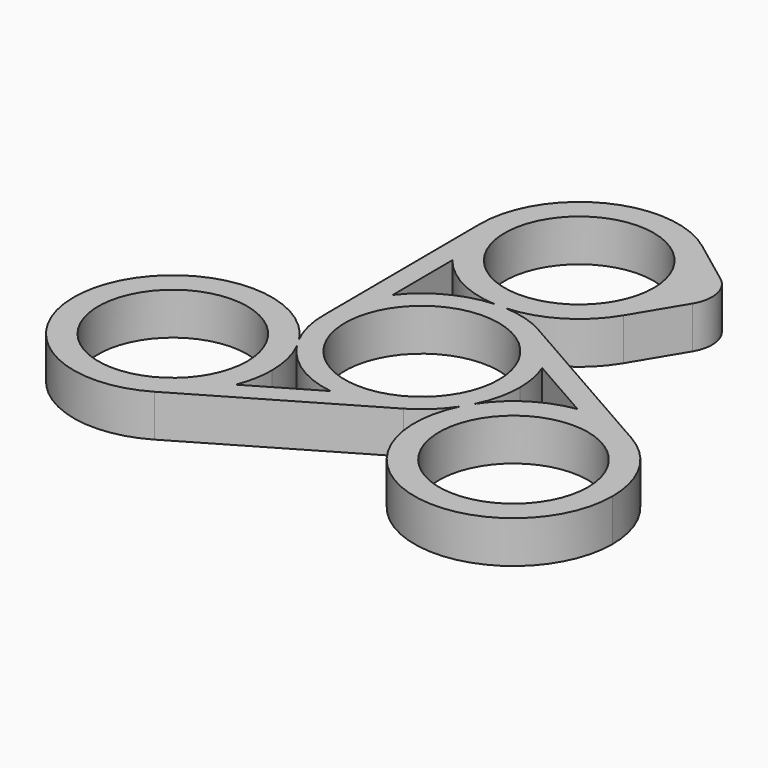
from build123d import *

# Parameters (mm, degrees)
F0_R     = 10.95
F0_R_2   = 10.6
F1_DEPTH = 6
F2_R     = 5


with BuildPart() as f1:
    # F0 (on Top) → F1 (new body)
    with BuildSketch(Plane.XY):
        with BuildLine():
            ThreePointArc((12.4777984827, -6.2375512043), (13.5769618994, -3.2044665053), (13.95, 0))
            ThreePointArc((13.95, 0), (13.6931728351, 2.6644920167), (12.932147999, 5.2308745094))
            ThreePointArc((12.932147999, 5.2308745094), (10.5018317529, 9.1822671401), (6.9101799774, 12.118247096))
            ThreePointArc((6.9101799774, 12.118247096), (3.977530702, 13.3709292689), (0.8370214411, 13.9248660714))
            ThreePointArc((0.8370214411, 13.9248660714), (0, 13.9), (-0.8370214411, 13.9248660714))
            ThreePointArc((-0.8370214411, 13.9248660714), (-6.4912873033, 12.3476997512), (-10.9961438792, 8.5841318599))
            ThreePointArc((-10.9961438792, 8.5841318599), (-13.2029923977, 4.5037197676), (-13.9497998232, -0.0747321429))
            ThreePointArc((-13.9497998232, -0.0747321429), (-13.5683297701, -3.2408220022), (-12.4777984827, -6.2375512043))
            ThreePointArc((-12.4777984827, -6.2375512043), (-12.0377531126, -6.95), (-11.6407770416, -7.6873148672))
            ThreePointArc((-11.6407770416, -7.6873148672), (-7.4477777849, -11.7954697264), (-1.9360037904, -13.8150059473))
            ThreePointArc((-1.9360037904, -13.8150059473), (2.7011607312, -13.6859866544), (7.0396198458, -12.0435149532))
            ThreePointArc((7.0396198458, -12.0435149532), (9.5907990681, -10.1301072667), (11.6407770416, -7.6873148672))
            ThreePointArc((11.6407770416, -7.6873148672), (12.0377531126, -6.95), (12.4777984827, -6.2375512043))
        make_face()
        Circle(F0_R, mode=Mode.SUBTRACT)
        with BuildLine():
            ThreePointArc((6.9101799774, 12.118247096), (10.5018317529, 9.1822671401), (12.932147999, 5.2308745094))
            Line((12.932147999, 5.2308745094), (22.1940121838, -0.0505121414))
            ThreePointArc((22.1940121838, -0.0505121414), (26.8561983982, -0.1431962176), (31.2331942939, -1.7514491718))
            Line((31.2331942939, -1.7514491718), (6.9101799774, 12.118247096))
        make_face()
        with BuildLine():
            ThreePointArc((22.1940121838, -0.0505121414), (16.67528741, -2.1065879373), (12.4777984827, -6.2375512043))
            ThreePointArc((12.4777984827, -6.2375512043), (12.0810543828, -6.975), (11.6407770416, -7.6873148672))
            ThreePointArc((11.6407770416, -7.6873148672), (21.0054007386, -27.7219144642), (38.348711306, -14))
            ThreePointArc((38.348711306, -14), (36.4407416974, -6.9173172501), (31.2331942939, -1.7514491718))
            ThreePointArc((31.2331942939, -1.7514491718), (26.8561983982, -0.1431962176), (22.1940121838, -0.0505121414))
        make_face()
        with Locations((24.248711306, -14)):
            Circle(F0_R_2, mode=Mode.SUBTRACT)
        with BuildLine():
            ThreePointArc((11.6407770416, -7.6873148672), (12.0810543828, -6.975), (12.4777984827, -6.2375512043))
            ThreePointArc((12.4777984827, -6.2375512043), (12.0377531126, -6.95), (11.6407770416, -7.6873148672))
        make_face()
        with BuildLine():
            ThreePointArc((-0.8370214411, 13.9248660714), (0, 13.9), (0.8370214411, 13.9248660714))
            ThreePointArc((0.8370214411, 13.9248660714), (0, 13.95), (-0.8370214411, 13.9248660714))
        make_face()
        with BuildLine():
            ThreePointArc((-0.8370214411, 13.9248660714), (0, 13.95), (0.8370214411, 13.9248660714))
            ThreePointArc((0.8370214411, 13.9248660714), (7.3062558034, 15.940620823), (12.0881437953, 20.7414340546))
            ThreePointArc((12.0881437953, 20.7414340546), (13.5877302651, 24.2338897729), (14.1, 28))
            ThreePointArc((14.1, 28), (12.6120042357, 34.3045498776), (8.4620781334, 39.2784411008))
            ThreePointArc((8.4620781334, 39.2784411008), (-6.338309536, 40.5950717436), (-14.0997976707, 27.9244642857))
            ThreePointArc((-14.0997976707, 27.9244642857), (-13.3040875478, 23.329747917), (-11.0532609603, 19.2458340121))
            ThreePointArc((-11.0532609603, 19.2458340121), (-6.5132847974, 15.4945163569), (-0.8370214411, 13.9248660714))
        make_face()
        with Locations((0, 28)):
            Circle(F0_R_2, mode=Mode.SUBTRACT)
        with BuildLine():
            Line((-17.1333966231, -26.1730151139), (7.0396198458, -12.0435149532))
            ThreePointArc((7.0396198458, -12.0435149532), (2.7011607312, -13.6859866544), (-1.9360037904, -13.8150059473))
            Line((-1.9360037904, -13.8150059473), (-11.1407508896, -19.1953222924))
            ThreePointArc((-11.1407508896, -19.1953222924), (-13.5521107613, -23.1865519531), (-17.1333966231, -26.1730151139))
        make_face()
        with BuildLine():
            ThreePointArc((14.1, 28), (13.5877302651, 24.2338897729), (12.0881437953, 20.7414340546))
            Line((12.0881437953, 20.7414340546), (18.6356199511, 31.6453555542))
            Line((18.6356199511, 31.6453555542), (8.4620781334, 39.2784411008))
            ThreePointArc((8.4620781334, 39.2784411008), (12.6120042357, 34.3045498776), (14.1, 28))
        make_face()
        with BuildLine():
            ThreePointArc((-12.4777984827, -6.2375512043), (-37.9792640143, -10.7934563276), (-17.1333966231, -26.1730151139))
            ThreePointArc((-17.1333966231, -26.1730151139), (-13.5521107613, -23.1865519531), (-11.1407508896, -19.1953222924))
            ThreePointArc((-11.1407508896, -19.1953222924), (-10.398941599, -16.64459431), (-10.148711306, -14))
            ThreePointArc((-10.148711306, -14), (-10.5267968417, -10.7566894326), (-11.6407770416, -7.6873148672))
            ThreePointArc((-11.6407770416, -7.6873148672), (-12.0810543828, -6.975), (-12.4777984827, -6.2375512043))
        make_face()
        with Locations((-24.248711306, -14)):
            Circle(F0_R_2, mode=Mode.SUBTRACT)
        with BuildLine():
            ThreePointArc((-13.9497998232, -0.0747321429), (-13.2029923977, 4.5037197676), (-10.9961438792, 8.5841318599))
            Line((-10.9961438792, 8.5841318599), (-11.0532609603, 19.2458340121))
            ThreePointArc((-11.0532609603, 19.2458340121), (-13.3040875478, 23.329747917), (-14.0997976707, 27.9244642857))
            Line((-14.0997976707, 27.9244642857), (-13.9497998232, -0.0747321429))
        make_face()
        with BuildLine():
            ThreePointArc((-12.4777984827, -6.2375512043), (-12.0810543828, -6.975), (-11.6407770416, -7.6873148672))
            ThreePointArc((-11.6407770416, -7.6873148672), (-12.0377531126, -6.95), (-12.4777984827, -6.2375512043))
        make_face()
    extrude(amount=F1_DEPTH)

    # F2
    f2_edges = [f1.edges().sort_by_distance(p)[0] for p in [
        (18.63562, 31.645356, 3),
    ]]
    fillet(f2_edges, radius=F2_R)


solid = f1.part
